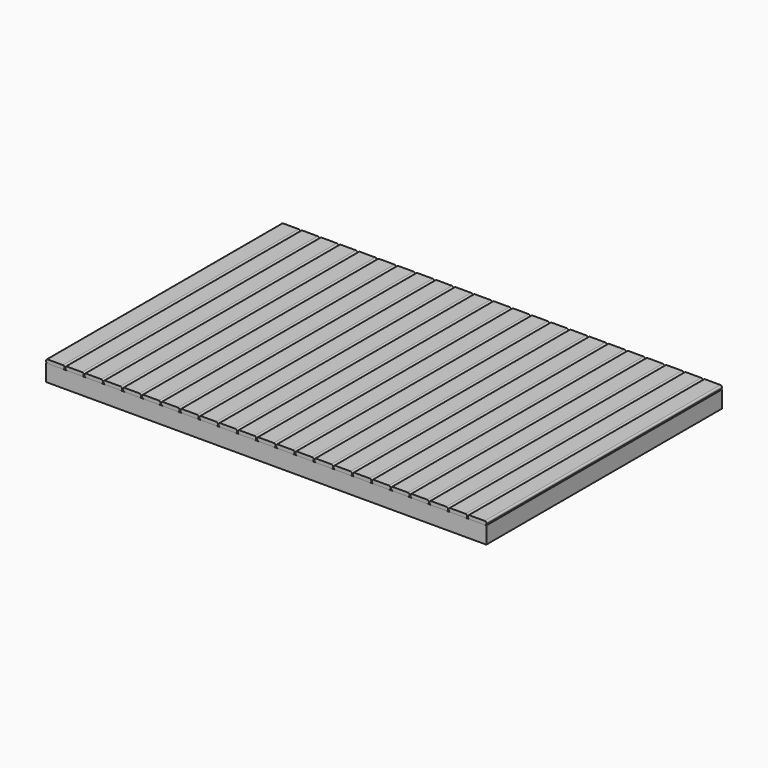
from build123d import *

# Parameters (mm, degrees)
F0_W     = 3568.7
F0_H     = 38.1
F1_DEPTH = 139.7
F3_DEPTH = 2438.4


with BuildPart() as f1:
    # F0 (on Top) → F1 (new body)
    with BuildSketch(Plane.XY):
        with Locations((0, 1200.15)):
            Rectangle(F0_W, F0_H)
        Polygon((-1784.35, 619.125), (-1784.35, 1181.1), (-1784.35, 1219.2), (-1822.45, 1219.2), (-1822.45, -1219.2), (-1784.35, -1219.2), (-1784.35, -1181.1), (-1784.35, -619.125), (-1784.35, -581.025), (-1784.35, -19.05), (-1784.35, 19.05), (-1784.35, 581.025), align=None)
        with Locations((0, 600.075)):
            Rectangle(F0_W, F0_H)
        Rectangle(F0_W, F0_H)
        with Locations((0, -600.075)):
            Rectangle(F0_W, F0_H)
        with Locations((0, -1200.15)):
            Rectangle(F0_W, F0_H)
        Polygon((1784.35, 1219.2), (1784.35, 1181.1), (1784.35, 619.125), (1784.35, 581.025), (1784.35, 19.05), (1784.35, -19.05), (1784.35, -581.025), (1784.35, -619.125), (1784.35, -1181.1), (1784.35, -1219.2), (1822.45, -1219.2), (1822.45, 1219.2), align=None)
    extrude(amount=F1_DEPTH)


with BuildPart() as f3:
    # F2 (on face) → F3 (new body)
    with BuildSketch(Plane.XZ.offset(1219.2)):
        with BuildLine():
            ThreePointArc((-1822.45, 152.4), (-1818.7302561211, 143.4197438789), (-1809.75, 139.7))
            Line((-1809.75, 139.7), (-1682.75, 139.7))
            ThreePointArc((-1682.75, 139.7), (-1673.7697438789, 143.4197438789), (-1670.05, 152.4))
            Line((-1670.05, 152.4), (-1670.05, 156.36875))
            ThreePointArc((-1670.05, 156.36875), (-1673.7697438789, 165.3490061211), (-1682.75, 169.06875))
            Line((-1682.75, 169.06875), (-1809.75, 169.06875))
            ThreePointArc((-1809.75, 169.06875), (-1818.7302561211, 165.3490061211), (-1822.45, 156.36875))
            Line((-1822.45, 156.36875), (-1822.45, 152.4))
        make_face()
    extrude(amount=-F3_DEPTH)


with BuildPart() as f3b:
    # F2 (on face) → F3, piece 2 (new body)
    with BuildSketch(Plane.XZ.offset(1219.2)):
        with BuildLine():
            ThreePointArc((-1663.7, 152.4), (-1659.9802561211, 143.4197438789), (-1651, 139.7))
            Line((-1651, 139.7), (-1524, 139.7))
            ThreePointArc((-1524, 139.7), (-1515.0197438789, 143.4197438789), (-1511.3, 152.4))
            Line((-1511.3, 152.4), (-1511.3, 156.36875))
            ThreePointArc((-1511.3, 156.36875), (-1515.0197438789, 165.3490061211), (-1524, 169.06875))
            Line((-1524, 169.06875), (-1651, 169.06875))
            ThreePointArc((-1651, 169.06875), (-1659.9802561211, 165.3490061211), (-1663.7, 156.36875))
            Line((-1663.7, 156.36875), (-1663.7, 152.4))
        make_face()
    extrude(amount=-F3_DEPTH)


with BuildPart() as f3c:
    # F2 (on face) → F3, piece 3 (new body)
    with BuildSketch(Plane.XZ.offset(1219.2)):
        with BuildLine():
            ThreePointArc((-1504.95, 152.4), (-1501.2302561211, 143.4197438789), (-1492.25, 139.7))
            Line((-1492.25, 139.7), (-1365.25, 139.7))
            ThreePointArc((-1365.25, 139.7), (-1356.2697438789, 143.4197438789), (-1352.55, 152.4))
            Line((-1352.55, 152.4), (-1352.55, 156.36875))
            ThreePointArc((-1352.55, 156.36875), (-1356.2697438789, 165.3490061211), (-1365.25, 169.06875))
            Line((-1365.25, 169.06875), (-1492.25, 169.06875))
            ThreePointArc((-1492.25, 169.06875), (-1501.2302561211, 165.3490061211), (-1504.95, 156.36875))
            Line((-1504.95, 156.36875), (-1504.95, 152.4))
        make_face()
    extrude(amount=-F3_DEPTH)


with BuildPart() as f3d:
    # F2 (on face) → F3, piece 4 (new body)
    with BuildSketch(Plane.XZ.offset(1219.2)):
        with BuildLine():
            Line((1682.75, 139.7), (1809.75, 139.7))
            ThreePointArc((1809.75, 139.7), (1818.7302561211, 143.4197438789), (1822.45, 152.4))
            Line((1822.45, 152.4), (1822.45, 156.36875))
            ThreePointArc((1822.45, 156.36875), (1818.7302561211, 165.3490061211), (1809.75, 169.06875))
            Line((1809.75, 169.06875), (1682.75, 169.06875))
            ThreePointArc((1682.75, 169.06875), (1673.7697438789, 165.3490061211), (1670.05, 156.36875))
            Line((1670.05, 156.36875), (1670.05, 152.4))
            ThreePointArc((1670.05, 152.4), (1673.7697438789, 143.4197438789), (1682.75, 139.7))
        make_face()
    extrude(amount=-F3_DEPTH)


with BuildPart() as f3e:
    # F2 (on face) → F3, piece 5 (new body)
    with BuildSketch(Plane.XZ.offset(1219.2)):
        with BuildLine():
            ThreePointArc((-1346.2, 152.4), (-1342.4802561211, 143.4197438789), (-1333.5, 139.7))
            Line((-1333.5, 139.7), (-1206.5, 139.7))
            ThreePointArc((-1206.5, 139.7), (-1197.5197438789, 143.4197438789), (-1193.8, 152.4))
            Line((-1193.8, 152.4), (-1193.8, 156.36875))
            ThreePointArc((-1193.8, 156.36875), (-1197.5197438789, 165.3490061211), (-1206.5, 169.06875))
            Line((-1206.5, 169.06875), (-1333.5, 169.06875))
            ThreePointArc((-1333.5, 169.06875), (-1342.4802561211, 165.3490061211), (-1346.2, 156.36875))
            Line((-1346.2, 156.36875), (-1346.2, 152.4))
        make_face()
    extrude(amount=-F3_DEPTH)


with BuildPart() as f3f:
    # F2 (on face) → F3, piece 6 (new body)
    with BuildSketch(Plane.XZ.offset(1219.2)):
        with BuildLine():
            Line((1524, 139.7), (1651, 139.7))
            ThreePointArc((1651, 139.7), (1659.9802561211, 143.4197438789), (1663.7, 152.4))
            Line((1663.7, 152.4), (1663.7, 156.36875))
            ThreePointArc((1663.7, 156.36875), (1659.9802561211, 165.3490061211), (1651, 169.06875))
            Line((1651, 169.06875), (1524, 169.06875))
            ThreePointArc((1524, 169.06875), (1515.0197438789, 165.3490061211), (1511.3, 156.36875))
            Line((1511.3, 156.36875), (1511.3, 152.4))
            ThreePointArc((1511.3, 152.4), (1515.0197438789, 143.4197438789), (1524, 139.7))
        make_face()
    extrude(amount=-F3_DEPTH)


with BuildPart() as f3g:
    # F2 (on face) → F3, piece 7 (new body)
    with BuildSketch(Plane.XZ.offset(1219.2)):
        with BuildLine():
            ThreePointArc((-1187.45, 152.4), (-1183.7302561211, 143.4197438789), (-1174.75, 139.7))
            Line((-1174.75, 139.7), (-1047.75, 139.7))
            ThreePointArc((-1047.75, 139.7), (-1038.7697438789, 143.4197438789), (-1035.05, 152.4))
            Line((-1035.05, 152.4), (-1035.05, 156.36875))
            ThreePointArc((-1035.05, 156.36875), (-1038.7697438789, 165.3490061211), (-1047.75, 169.06875))
            Line((-1047.75, 169.06875), (-1174.75, 169.06875))
            ThreePointArc((-1174.75, 169.06875), (-1183.7302561211, 165.3490061211), (-1187.45, 156.36875))
            Line((-1187.45, 156.36875), (-1187.45, 152.4))
        make_face()
    extrude(amount=-F3_DEPTH)


with BuildPart() as f3h:
    # F2 (on face) → F3, piece 8 (new body)
    with BuildSketch(Plane.XZ.offset(1219.2)):
        with BuildLine():
            Line((1365.25, 139.7), (1492.25, 139.7))
            ThreePointArc((1492.25, 139.7), (1501.2302561211, 143.4197438789), (1504.95, 152.4))
            Line((1504.95, 152.4), (1504.95, 156.36875))
            ThreePointArc((1504.95, 156.36875), (1501.2302561211, 165.3490061211), (1492.25, 169.06875))
            Line((1492.25, 169.06875), (1365.25, 169.06875))
            ThreePointArc((1365.25, 169.06875), (1356.2697438789, 165.3490061211), (1352.55, 156.36875))
            Line((1352.55, 156.36875), (1352.55, 152.4))
            ThreePointArc((1352.55, 152.4), (1356.2697438789, 143.4197438789), (1365.25, 139.7))
        make_face()
    extrude(amount=-F3_DEPTH)


with BuildPart() as f3i:
    # F2 (on face) → F3, piece 9 (new body)
    with BuildSketch(Plane.XZ.offset(1219.2)):
        with BuildLine():
            ThreePointArc((-1028.7, 152.4), (-1024.9802561211, 143.4197438789), (-1016, 139.7))
            Line((-1016, 139.7), (-889, 139.7))
            ThreePointArc((-889, 139.7), (-880.0197438789, 143.4197438789), (-876.3, 152.4))
            Line((-876.3, 152.4), (-876.3, 156.36875))
            ThreePointArc((-876.3, 156.36875), (-880.0197438789, 165.3490061211), (-889, 169.06875))
            Line((-889, 169.06875), (-1016, 169.06875))
            ThreePointArc((-1016, 169.06875), (-1024.9802561211, 165.3490061211), (-1028.7, 156.36875))
            Line((-1028.7, 156.36875), (-1028.7, 152.4))
        make_face()
    extrude(amount=-F3_DEPTH)


with BuildPart() as f3j:
    # F2 (on face) → F3, piece 10 (new body)
    with BuildSketch(Plane.XZ.offset(1219.2)):
        with BuildLine():
            Line((1206.5, 139.7), (1333.5, 139.7))
            ThreePointArc((1333.5, 139.7), (1342.4802561211, 143.4197438789), (1346.2, 152.4))
            Line((1346.2, 152.4), (1346.2, 156.36875))
            ThreePointArc((1346.2, 156.36875), (1342.4802561211, 165.3490061211), (1333.5, 169.06875))
            Line((1333.5, 169.06875), (1206.5, 169.06875))
            ThreePointArc((1206.5, 169.06875), (1197.5197438789, 165.3490061211), (1193.8, 156.36875))
            Line((1193.8, 156.36875), (1193.8, 152.4))
            ThreePointArc((1193.8, 152.4), (1197.5197438789, 143.4197438789), (1206.5, 139.7))
        make_face()
    extrude(amount=-F3_DEPTH)


with BuildPart() as f3k:
    # F2 (on face) → F3, piece 11 (new body)
    with BuildSketch(Plane.XZ.offset(1219.2)):
        with BuildLine():
            ThreePointArc((-869.95, 152.4), (-866.2302561211, 143.4197438789), (-857.25, 139.7))
            Line((-857.25, 139.7), (-730.25, 139.7))
            ThreePointArc((-730.25, 139.7), (-721.2697438789, 143.4197438789), (-717.55, 152.4))
            Line((-717.55, 152.4), (-717.55, 156.36875))
            ThreePointArc((-717.55, 156.36875), (-721.2697438789, 165.3490061211), (-730.25, 169.06875))
            Line((-730.25, 169.06875), (-857.25, 169.06875))
            ThreePointArc((-857.25, 169.06875), (-866.2302561211, 165.3490061211), (-869.95, 156.36875))
            Line((-869.95, 156.36875), (-869.95, 152.4))
        make_face()
    extrude(amount=-F3_DEPTH)


with BuildPart() as f3l:
    # F2 (on face) → F3, piece 12 (new body)
    with BuildSketch(Plane.XZ.offset(1219.2)):
        with BuildLine():
            Line((1047.75, 139.7), (1174.75, 139.7))
            ThreePointArc((1174.75, 139.7), (1183.7302561211, 143.4197438789), (1187.45, 152.4))
            Line((1187.45, 152.4), (1187.45, 156.36875))
            ThreePointArc((1187.45, 156.36875), (1183.7302561211, 165.3490061211), (1174.75, 169.06875))
            Line((1174.75, 169.06875), (1047.75, 169.06875))
            ThreePointArc((1047.75, 169.06875), (1038.7697438789, 165.3490061211), (1035.05, 156.36875))
            Line((1035.05, 156.36875), (1035.05, 152.4))
            ThreePointArc((1035.05, 152.4), (1038.7697438789, 143.4197438789), (1047.75, 139.7))
        make_face()
    extrude(amount=-F3_DEPTH)


with BuildPart() as f3m:
    # F2 (on face) → F3, piece 13 (new body)
    with BuildSketch(Plane.XZ.offset(1219.2)):
        with BuildLine():
            ThreePointArc((-711.2, 152.4), (-707.4802561211, 143.4197438789), (-698.5, 139.7))
            Line((-698.5, 139.7), (-571.5, 139.7))
            ThreePointArc((-571.5, 139.7), (-562.5197438789, 143.4197438789), (-558.8, 152.4))
            Line((-558.8, 152.4), (-558.8, 156.36875))
            ThreePointArc((-558.8, 156.36875), (-562.5197438789, 165.3490061211), (-571.5, 169.06875))
            Line((-571.5, 169.06875), (-698.5, 169.06875))
            ThreePointArc((-698.5, 169.06875), (-707.4802561211, 165.3490061211), (-711.2, 156.36875))
            Line((-711.2, 156.36875), (-711.2, 152.4))
        make_face()
    extrude(amount=-F3_DEPTH)


with BuildPart() as f3n:
    # F2 (on face) → F3, piece 14 (new body)
    with BuildSketch(Plane.XZ.offset(1219.2)):
        with BuildLine():
            Line((889, 139.7), (1016, 139.7))
            ThreePointArc((1016, 139.7), (1024.9802561211, 143.4197438789), (1028.7, 152.4))
            Line((1028.7, 152.4), (1028.7, 156.36875))
            ThreePointArc((1028.7, 156.36875), (1024.9802561211, 165.3490061211), (1016, 169.06875))
            Line((1016, 169.06875), (889, 169.06875))
            ThreePointArc((889, 169.06875), (880.0197438789, 165.3490061211), (876.3, 156.36875))
            Line((876.3, 156.36875), (876.3, 152.4))
            ThreePointArc((876.3, 152.4), (880.0197438789, 143.4197438789), (889, 139.7))
        make_face()
    extrude(amount=-F3_DEPTH)


with BuildPart() as f3o:
    # F2 (on face) → F3, piece 15 (new body)
    with BuildSketch(Plane.XZ.offset(1219.2)):
        with BuildLine():
            ThreePointArc((-552.45, 152.4), (-548.7302561211, 143.4197438789), (-539.75, 139.7))
            Line((-539.75, 139.7), (-412.75, 139.7))
            ThreePointArc((-412.75, 139.7), (-403.7697438789, 143.4197438789), (-400.05, 152.4))
            Line((-400.05, 152.4), (-400.05, 156.36875))
            ThreePointArc((-400.05, 156.36875), (-403.7697438789, 165.3490061211), (-412.75, 169.06875))
            Line((-412.75, 169.06875), (-539.75, 169.06875))
            ThreePointArc((-539.75, 169.06875), (-548.7302561211, 165.3490061211), (-552.45, 156.36875))
            Line((-552.45, 156.36875), (-552.45, 152.4))
        make_face()
    extrude(amount=-F3_DEPTH)


with BuildPart() as f3p:
    # F2 (on face) → F3, piece 16 (new body)
    with BuildSketch(Plane.XZ.offset(1219.2)):
        with BuildLine():
            Line((730.25, 139.7), (857.25, 139.7))
            ThreePointArc((857.25, 139.7), (866.2302561211, 143.4197438789), (869.95, 152.4))
            Line((869.95, 152.4), (869.95, 156.36875))
            ThreePointArc((869.95, 156.36875), (866.2302561211, 165.3490061211), (857.25, 169.06875))
            Line((857.25, 169.06875), (730.25, 169.06875))
            ThreePointArc((730.25, 169.06875), (721.2697438789, 165.3490061211), (717.55, 156.36875))
            Line((717.55, 156.36875), (717.55, 152.4))
            ThreePointArc((717.55, 152.4), (721.2697438789, 143.4197438789), (730.25, 139.7))
        make_face()
    extrude(amount=-F3_DEPTH)


with BuildPart() as f3q:
    # F2 (on face) → F3, piece 17 (new body)
    with BuildSketch(Plane.XZ.offset(1219.2)):
        with BuildLine():
            ThreePointArc((-393.7, 152.4), (-389.9802561211, 143.4197438789), (-381, 139.7))
            Line((-381, 139.7), (-254, 139.7))
            ThreePointArc((-254, 139.7), (-245.0197438789, 143.4197438789), (-241.3, 152.4))
            Line((-241.3, 152.4), (-241.3, 156.36875))
            ThreePointArc((-241.3, 156.36875), (-245.0197438789, 165.3490061211), (-254, 169.06875))
            Line((-254, 169.06875), (-381, 169.06875))
            ThreePointArc((-381, 169.06875), (-389.9802561211, 165.3490061211), (-393.7, 156.36875))
            Line((-393.7, 156.36875), (-393.7, 152.4))
        make_face()
    extrude(amount=-F3_DEPTH)


with BuildPart() as f3r:
    # F2 (on face) → F3, piece 18 (new body)
    with BuildSketch(Plane.XZ.offset(1219.2)):
        with BuildLine():
            Line((571.5, 139.7), (698.5, 139.7))
            ThreePointArc((698.5, 139.7), (707.4802561211, 143.4197438789), (711.2, 152.4))
            Line((711.2, 152.4), (711.2, 156.36875))
            ThreePointArc((711.2, 156.36875), (707.4802561211, 165.3490061211), (698.5, 169.06875))
            Line((698.5, 169.06875), (571.5, 169.06875))
            ThreePointArc((571.5, 169.06875), (562.5197438789, 165.3490061211), (558.8, 156.36875))
            Line((558.8, 156.36875), (558.8, 152.4))
            ThreePointArc((558.8, 152.4), (562.5197438789, 143.4197438789), (571.5, 139.7))
        make_face()
    extrude(amount=-F3_DEPTH)


with BuildPart() as f3s:
    # F2 (on face) → F3, piece 19 (new body)
    with BuildSketch(Plane.XZ.offset(1219.2)):
        with BuildLine():
            ThreePointArc((-234.95, 152.4), (-231.2302561211, 143.4197438789), (-222.25, 139.7))
            Line((-222.25, 139.7), (-95.25, 139.7))
            ThreePointArc((-95.25, 139.7), (-86.2697438789, 143.4197438789), (-82.55, 152.4))
            Line((-82.55, 152.4), (-82.55, 156.36875))
            ThreePointArc((-82.55, 156.36875), (-86.2697438789, 165.3490061211), (-95.25, 169.06875))
            Line((-95.25, 169.06875), (-222.25, 169.06875))
            ThreePointArc((-222.25, 169.06875), (-231.2302561211, 165.3490061211), (-234.95, 156.36875))
            Line((-234.95, 156.36875), (-234.95, 152.4))
        make_face()
    extrude(amount=-F3_DEPTH)


with BuildPart() as f3t:
    # F2 (on face) → F3, piece 20 (new body)
    with BuildSketch(Plane.XZ.offset(1219.2)):
        with BuildLine():
            Line((412.75, 139.7), (539.75, 139.7))
            ThreePointArc((539.75, 139.7), (548.7302561211, 143.4197438789), (552.45, 152.4))
            Line((552.45, 152.4), (552.45, 156.36875))
            ThreePointArc((552.45, 156.36875), (548.7302561211, 165.3490061211), (539.75, 169.06875))
            Line((539.75, 169.06875), (412.75, 169.06875))
            ThreePointArc((412.75, 169.06875), (403.7697438789, 165.3490061211), (400.05, 156.36875))
            Line((400.05, 156.36875), (400.05, 152.4))
            ThreePointArc((400.05, 152.4), (403.7697438789, 143.4197438789), (412.75, 139.7))
        make_face()
    extrude(amount=-F3_DEPTH)


with BuildPart() as f3u:
    # F2 (on face) → F3, piece 21 (new body)
    with BuildSketch(Plane.XZ.offset(1219.2)):
        with BuildLine():
            ThreePointArc((-76.2, 152.4), (-72.4802561211, 143.4197438789), (-63.5, 139.7))
            Line((-63.5, 139.7), (63.5, 139.7))
            ThreePointArc((63.5, 139.7), (72.4802561211, 143.4197438789), (76.2, 152.4))
            Line((76.2, 152.4), (76.2, 156.36875))
            ThreePointArc((76.2, 156.36875), (72.4802561211, 165.3490061211), (63.5, 169.06875))
            Line((63.5, 169.06875), (-63.5, 169.06875))
            ThreePointArc((-63.5, 169.06875), (-72.4802561211, 165.3490061211), (-76.2, 156.36875))
            Line((-76.2, 156.36875), (-76.2, 152.4))
        make_face()
    extrude(amount=-F3_DEPTH)


with BuildPart() as f3v:
    # F2 (on face) → F3, piece 22 (new body)
    with BuildSketch(Plane.XZ.offset(1219.2)):
        with BuildLine():
            Line((254, 139.7), (381, 139.7))
            ThreePointArc((381, 139.7), (389.9802561211, 143.4197438789), (393.7, 152.4))
            Line((393.7, 152.4), (393.7, 156.36875))
            ThreePointArc((393.7, 156.36875), (389.9802561211, 165.3490061211), (381, 169.06875))
            Line((381, 169.06875), (254, 169.06875))
            ThreePointArc((254, 169.06875), (245.0197438789, 165.3490061211), (241.3, 156.36875))
            Line((241.3, 156.36875), (241.3, 152.4))
            ThreePointArc((241.3, 152.4), (245.0197438789, 143.4197438789), (254, 139.7))
        make_face()
    extrude(amount=-F3_DEPTH)


with BuildPart() as f3w:
    # F2 (on face) → F3, piece 23 (new body)
    with BuildSketch(Plane.XZ.offset(1219.2)):
        with BuildLine():
            ThreePointArc((82.55, 152.4), (86.2697438789, 143.4197438789), (95.25, 139.7))
            Line((95.25, 139.7), (222.25, 139.7))
            ThreePointArc((222.25, 139.7), (231.2302561211, 143.4197438789), (234.95, 152.4))
            Line((234.95, 152.4), (234.95, 156.36875))
            ThreePointArc((234.95, 156.36875), (231.2302561211, 165.3490061211), (222.25, 169.06875))
            Line((222.25, 169.06875), (95.25, 169.06875))
            ThreePointArc((95.25, 169.06875), (86.2697438789, 165.3490061211), (82.55, 156.36875))
            Line((82.55, 156.36875), (82.55, 152.4))
        make_face()
    extrude(amount=-F3_DEPTH)


solid = Compound([f1.part, f3.part, f3b.part, f3c.part, f3d.part, f3e.part, f3f.part, f3g.part, f3h.part, f3i.part, f3j.part, f3k.part, f3l.part, f3m.part, f3n.part, f3o.part, f3p.part, f3q.part, f3r.part, f3s.part, f3t.part, f3u.part, f3v.part, f3w.part])
